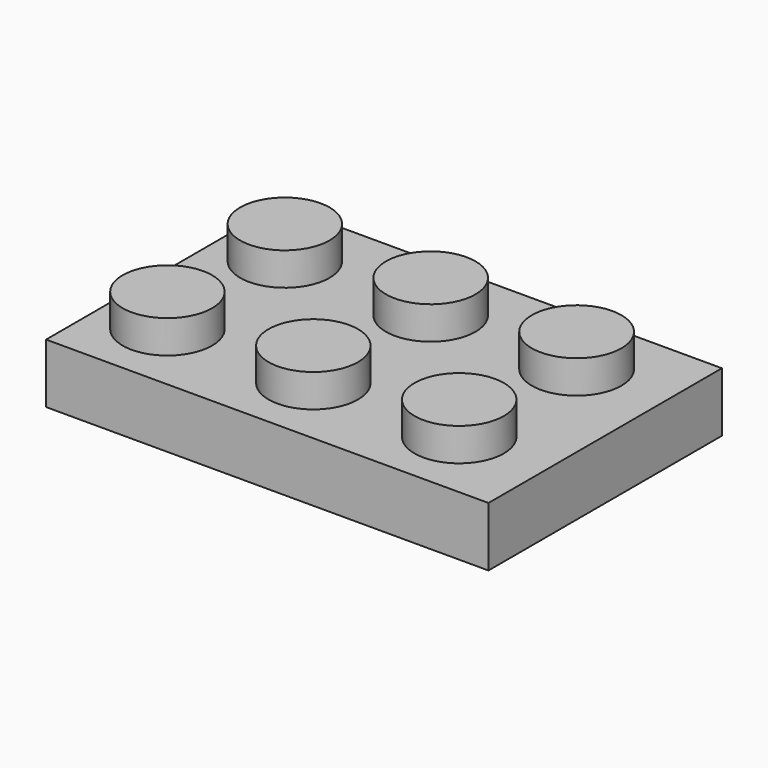
from build123d import *

# Parameters (mm, degrees)
F0_W      = 23.876
F0_H      = 15.748
F1_DEPTH  = 3.20802
F2_R      = 2.413
F3_DEPTH  = 1.778
F2_R_2    = 2.4164208991
F4_DEPTH  = 1.778
F2_R_3    = 2.4201182345
F5_DEPTH  = 1.778
F6_DEPTH  = 1.778
F7_DEPTH  = 1.778
F8_DEPTH  = 1.778
F9_T      = -1.778
F10_R     = 3.2385
F10_R_2   = 2.6416
F11_DEPTH = 3.06898


# Not quite as in the source:
# - a feature names something its author has since deleted; it is built from what else it names


with BuildPart() as f1:
    # F0 (on Top) → F1 (new body)
    with BuildSketch(Plane.XY):
        with Locations((11.938, 7.874)):
            Rectangle(F0_W, F0_H)
    extrude(amount=F1_DEPTH)

    # F2 (on face) → F3 (join)
    with BuildSketch(Plane.XY.offset(3.20802)):
        with Locations((3.3980837251, 11.858843371)):
            Circle(F2_R)
    extrude(amount=F3_DEPTH)

    # F2 (on face) → F4 (join)
    with BuildSketch(Plane.XY.offset(3.20802)):
        with Locations((11.2720837251, 11.858843371)):
            Circle(F2_R_2)
    extrude(amount=F4_DEPTH)

    # F2 (on face) → F5 (join)
    with BuildSketch(Plane.XY.offset(3.20802)):
        with Locations((19.1460837251, 11.858843371)):
            Circle(F2_R_3)
    extrude(amount=F5_DEPTH)

    # F2 (on face) → F6 (join)
    with BuildSketch(Plane.XY.offset(3.20802)):
        with Locations((3.3980837251, 3.9364123053)):
            Circle(F2_R)
    extrude(amount=F6_DEPTH)

    # F2 (on face) → F7 (join)
    with BuildSketch(Plane.XY.offset(3.20802)):
        with Locations((11.2720837251, 3.9364123053)):
            Circle(F2_R)
    extrude(amount=F7_DEPTH)

    # F2 (on face) → F8 (join)
    with BuildSketch(Plane.XY.offset(3.20802)):
        with Locations((19.1460837251, 3.9364123053)):
            Circle(F2_R)
    extrude(amount=F8_DEPTH)

    # F9
    f9_openings = [f1.faces().sort_by_distance(p)[0] for p in [
        (11.938, 7.874, 0),
    ]]
    offset(amount=F9_T, openings=f9_openings, kind=Kind.INTERSECTION)

    # F10 (on face) → F11 (join)
    with BuildSketch(Plane.XY):
        with BuildLine():
            ThreePointArc((4.1275, 7.5388690457), (7.366, 4.3003690457), (10.6045, 7.5388690457))
            ThreePointArc((10.6045, 7.5388690457), (7.366, 10.7773690457), (4.1275, 7.5388690457))
        make_face()
        with BuildLine():
            ThreePointArc((10.0076, 7.5388690457), (7.366, 4.8972690457), (4.7244, 7.5388690457))
            ThreePointArc((4.7244, 7.5388690457), (7.366, 10.1804690457), (10.0076, 7.5388690457))
        make_face(mode=Mode.SUBTRACT)
        with Locations((15.24, 7.5388690457)):
            Circle(F10_R)
        with Locations((15.24, 7.5388690457)):
            Circle(F10_R_2, mode=Mode.SUBTRACT)
    extrude(amount=F11_DEPTH)


solid = f1.part
